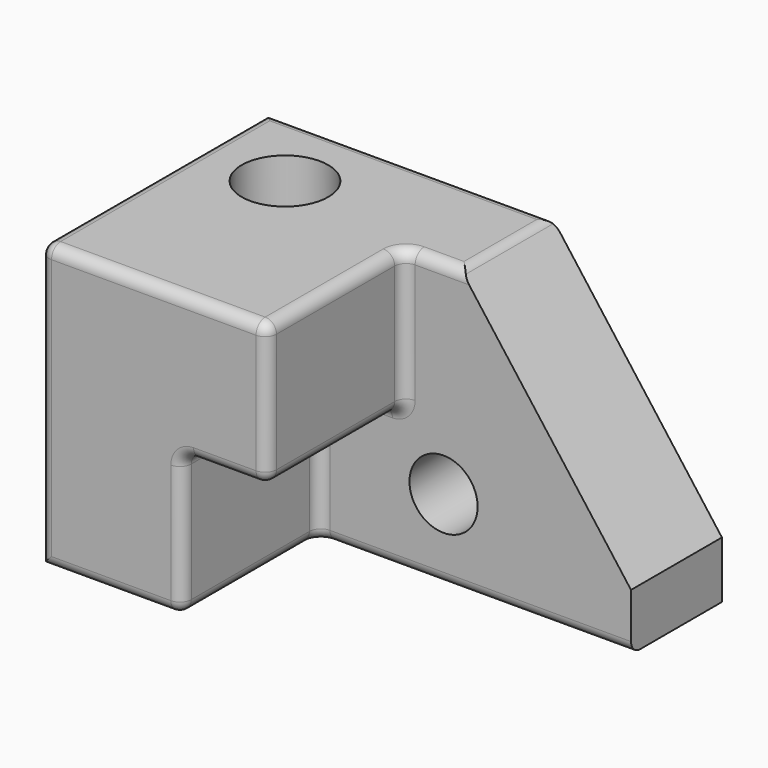
from build123d import *

# Parameters (mm, degrees)
F0_W     = 203.2
F0_H     = 127
F1_DEPTH = 127
F3_DEPTH = 76.2
F4_SIZE2 = 101.6
F4_SIZE  = 76.2
F5_R     = 5.08
F6_R     = 15.24
F7_DEPTH = 50.8
F8_R     = 19.349676851
F9_DEPTH = 127


with BuildPart() as f1:
    # F0 (on Front) → F1 (new body)
    with BuildSketch(Plane.XZ):
        with Locations((38.9206162602, 27.6787289854)):
            Rectangle(F0_W, F0_H)
    extrude(amount=F1_DEPTH)

    # F2 (on face) → F3 (cut)
    with BuildSketch(Plane.XZ.offset(127)):
        Polygon((38.9206162602, 27.6787289854), (0.8206162602, 27.6787289854), (0.8206162602, -35.8212710146), (140.5206162602, -35.8212710146), (140.5206162602, 91.1787289854), (38.9206162602, 91.1787289854), align=None)
    extrude(amount=-F3_DEPTH, mode=Mode.SUBTRACT)

    # F4
    f4_edges = [f1.edges().sort_by_distance(p)[0] for p in [
        (140.520616, -25.4, 91.178729),
    ]]
    f4_side = f1.faces().sort_by_distance((17.149188, -52.614286, 91.178729))[0]
    chamfer(f4_edges, length=F4_SIZE, length2=F4_SIZE2, reference=f4_side)

    # F5
    f5_edges = [f1.edges().sort_by_distance(p)[0] for p in [
        (-11.879384, -127, 91.178729),
        (38.920616, -127, 59.428729),
        (19.870616, -127, 27.678729),
        (0.820616, -127, -4.071271),
        (38.920616, -88.9, 27.678729),
        (-62.679384, -127, 27.678729),
        (0.820616, -88.9, 27.678729),
        (0.820616, -88.9, -35.821271),
        (0.820616, -50.8, -4.071271),
        (38.920616, -50.8, 59.428729),
        (38.920616, -88.9, 91.178729),
        (0.820616, 0, 91.178729),
        (64.320616, -25.4, 91.178729),
        (-62.679384, -63.5, 91.178729),
        (51.620616, -50.8, 91.178729),
        (-30.929384, -127, -35.821271),
        (70.670616, -50.8, -35.821271),
        (19.870616, -50.8, 27.678729),
    ]]
    fillet(f5_edges, radius=F5_R)

    # F6 (on face) → F7 (cut, through all)
    with BuildSketch(Plane.XZ.offset(50.8)):
        with Locations((56.7006162602, 0)):
            Circle(F6_R)
    extrude(amount=-F7_DEPTH, mode=Mode.SUBTRACT)

    # F8 (on face) → F9 (cut, through all)
    with BuildSketch(Plane.XY.offset(91.1787289854)):
        with Locations((-25.0357538462, -37.260428071)):
            Circle(F8_R)
    extrude(amount=-F9_DEPTH, mode=Mode.SUBTRACT)


solid = f1.part
